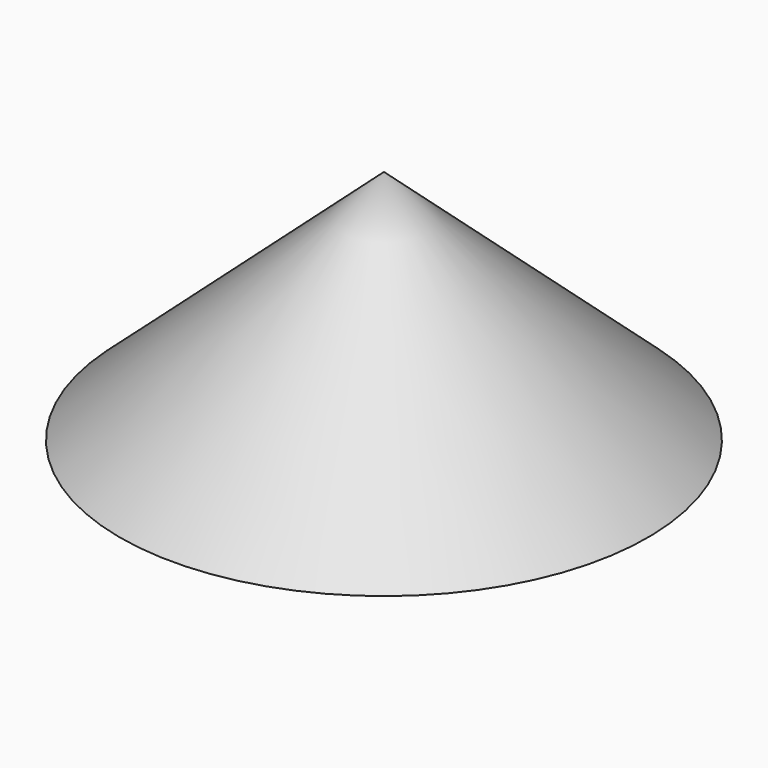
from build123d import *


# Not quite as in the source:
# - the program builds the solid bodies; features that only make, move or delete a surface that nothing else refers to are left out


with BuildPart() as f1:
    # F0 (on Right) → F1 (revolve)
    with BuildSketch(Plane.YZ):
        Polygon((0, 0), (-35.5558055322, 31.8025350571), (-35.5558055322, 0), align=None)
    revolve(axis=Axis((0, -35.5558055322, 15.9012675285), (0, 0, -1)))


solid = f1.part
